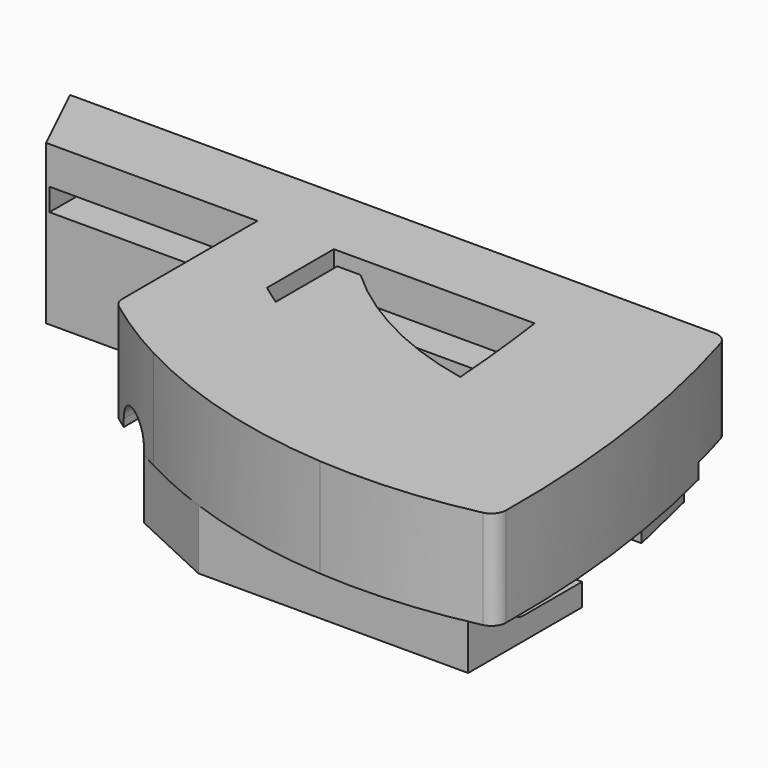
from build123d import *

# Parameters (mm, degrees)
F1_DEPTH  = 13.2
F3_DEPTH  = 8
F5_DEPTH  = 88.4390001176
F7_DEPTH  = 48.4308042409
F6_W      = 77
F6_H      = 3
F8_DEPTH  = 12.8
F9_R      = 5
F10_R     = 2
F12_DEPTH = 2
F13_W     = 40.65
F13_H     = 3
F13_W_2   = 12.25
F14_DEPTH = 23.0683441528


# Not quite as in the source:
# - a feature names something its author has since deleted; it is built from what else it names


with BuildPart() as f1:
    # F0 (on Top) → F1 (new body)
    with BuildSketch(Plane.XY):
        with BuildLine():
            Line((-3.2, -10), (4.8, -10))
            Line((4.8, -10), (25, -10))
            Line((25, -10), (25, -33.5))
            ThreePointArc((25, -33.5), (29.9617064043, -36.9938363193), (35.2, -40.0574457714))
            Line((35.2, -40.0574457714), (35.2, -21.1564938874))
            Line((35.2, -21.1564938874), (35.2, -10))
            Line((35.2, -10), (62, -10))
            ThreePointArc((62, -10), (62.8699868465, -17.1376907215), (63.5062507441, -24.3))
            ThreePointArc((63.5062507441, -24.3), (63.7566330876, -28.252847646), (63.9358126513, -32.2095622573))
            ThreePointArc((63.9358126513, -32.2095622573), (64.0273561468, -35.3542873695), (64.0739210442, -38.5))
            ThreePointArc((64.0739210442, -38.5), (64.0571349812, -43.3799777622), (63.9321127792, -48.258382643))
            ThreePointArc((63.9321127792, -48.258382643), (75.0391386854, -48.167385668), (86, -46.3691019944))
            ThreePointArc((86, -46.3691019944), (84.6340109104, -22.9204511896), (79.5, 0))
            Line((79.5, 0), (0, 0))
            Line((0, 0), (-8, 0))
            Line((-8, 0), (-3.2, -10))
        make_face()
        with BuildLine():
            Line((35.2, -21.1564938874), (35.2, -40.0574457714))
            ThreePointArc((35.2, -40.0574457714), (49.1359582734, -45.6647697988), (63.9321127792, -48.258382643))
            ThreePointArc((63.9321127792, -48.258382643), (64.0571349812, -43.3799777622), (64.0739210442, -38.5))
            ThreePointArc((64.0739210442, -38.5), (50.2282447294, -34.8385677857), (37.9, -27.55))
            Line((37.9, -27.55), (37.9, -23.0683441528))
            ThreePointArc((37.9, -23.0683441528), (36.5358784648, -22.1323620803), (35.2, -21.1564938874))
        make_face()
        with BuildLine():
            Line((37.9, -12.8), (37.9, -23.0683441528))
            ThreePointArc((37.9, -23.0683441528), (50.346051903, -29.2676961626), (63.9358126513, -32.2095622573))
            ThreePointArc((63.9358126513, -32.2095622573), (63.7566330876, -28.252847646), (63.5062507441, -24.3))
            ThreePointArc((63.5062507441, -24.3), (51.465613735, -20.0912116842), (41, -12.8))
            Line((41, -12.8), (37.9, -12.8))
        make_face()
        with BuildLine():
            ThreePointArc((63.9358126513, -32.2095622573), (50.346051903, -29.2676961626), (37.9, -23.0683441528))
            Line((37.9, -23.0683441528), (37.9, -27.55))
            ThreePointArc((37.9, -27.55), (50.2282447294, -34.8385677857), (64.0739210442, -38.5))
            ThreePointArc((64.0739210442, -38.5), (64.0273561468, -35.3542873695), (63.9358126513, -32.2095622573))
        make_face()
    extrude(amount=-F1_DEPTH)

    # F2 (on face) → F3 (join)
    with BuildSketch(Plane(origin=(0, 0, -13.2), x_dir=(1, 0, 0), z_dir=(0, 0, -1))):
        Polygon((0.35, 0), (27.35, 0), (27.35, 10), (25, 10), (-3.2, 10), (-8, 0), align=None)
        Polygon((32.85, 10), (32.85, 0), (73.9, 0), (76.2576692783, 10), (62, 10), (35.2, 10), align=None)
        Polygon((32.85, 25.1478344245), (80.4380001176, 25.1478344245), (80.4380001176, 44.1478344245), (44.4380001176, 44.1478344245), (32.85, 38.7561702211), align=None)
    extrude(amount=F3_DEPTH)

    # F4 (on face) → F5 (cut, through all)
    with BuildSketch(Plane.YZ.offset(80.4380001176)):
        with BuildLine():
            Line((0, -18.2), (0, -13.2))
            Line((0, -13.2), (-4.85, -13.2))
            ThreePointArc((-4.85, -13.2), (-7.35, -15.7), (-4.85, -18.2))
            Line((-4.85, -18.2), (0, -18.2))
        make_face()
        with BuildLine():
            Line((-34.85, -18.2), (-30, -18.2))
            Line((-30, -18.2), (-25.1478344245, -18.2))
            Line((-25.1478344245, -18.2), (-25.1478344245, -13.2))
            Line((-25.1478344245, -13.2), (-30, -13.2))
            Line((-30, -13.2), (-34.85, -13.2))
            ThreePointArc((-34.85, -13.2), (-37.35, -15.7), (-34.85, -18.2))
        make_face()
    extrude(amount=-F5_DEPTH, mode=Mode.SUBTRACT)

    # F6 (on face) → F7 (cut, through all)
    with BuildSketch(Plane(origin=(0, 0, 0), x_dir=(-1, 0, 0), z_dir=(0, 1, 0))):
        with BuildLine():
            Line((-32.85, -13.2), (-27.35, -13.2))
            Line((-27.35, -13.2), (-27.35, -12.2))
            ThreePointArc((-27.35, -12.2), (-30.1, -9.45), (-32.85, -12.2))
            Line((-32.85, -12.2), (-32.85, -13.2))
        make_face()
    extrude(amount=-F7_DEPTH, mode=Mode.SUBTRACT)

    # F6 (on face) → F8 (cut, through all)
    with BuildSketch(Plane(origin=(0, 0, 0), x_dir=(-1, 0, 0), z_dir=(0, 1, 0))):
        with Locations((-35.75, -6.5)):
            Rectangle(F6_W, F6_H)
    extrude(amount=-F8_DEPTH, mode=Mode.SUBTRACT)

    # F9
    f9_edges = [f1.edges().sort_by_distance(p)[0] for p in [
        (69.128835, -10, -13.2),
        (26.175, -10, -13.2),
    ]]
    fillet(f9_edges, radius=F9_R)

    # F10
    f10_edges = [f1.edges().sort_by_distance(p)[0] for p in [
        (86, -46.369102, -6.6),
        (79.5, 0, -6.6),
        (25, -33.5, -6.6),
    ]]
    fillet(f10_edges, radius=F10_R)

    # F11 (on face) → F12 (cut)
    with BuildSketch(Plane(origin=(0, 0, -13.2), x_dir=(1, 0, 0), z_dir=(0, 0, -1))):
        with BuildLine():
            Line((73.4852175089, 0), (78.0194737362, 0))
            ThreePointArc((78.0194737362, 0), (79.2135753482, 0.39559315), (79.9352985421, 1.4258786598))
            ThreePointArc((79.9352985421, 1.4258786598), (80.7380621658, 4.2052082165), (81.4852175089, 7))
            Line((81.4852175089, 7), (75.5503684948, 7))
            Line((75.5503684948, 7), (75.0434696, 4.85))
            Line((75.0434696, 4.85), (74.9160721206, 4.85))
            Line((74.9160721206, 4.85), (73.4852175089, 0))
        make_face()
    extrude(amount=-F12_DEPTH, mode=Mode.SUBTRACT)

    # F13 (on face) → F14 (cut, through all)
    with BuildSketch(Plane(origin=(0, 0, 0), x_dir=(-1, 0, 0), z_dir=(0, 1, 0))):
        with Locations((-17.575, -6.5)):
            Rectangle(F13_W, F13_H)
        with Locations((-68.125, -6.5)):
            Rectangle(F13_W_2, F13_H)
    extrude(amount=-F14_DEPTH, mode=Mode.SUBTRACT)


solid = f1.part
